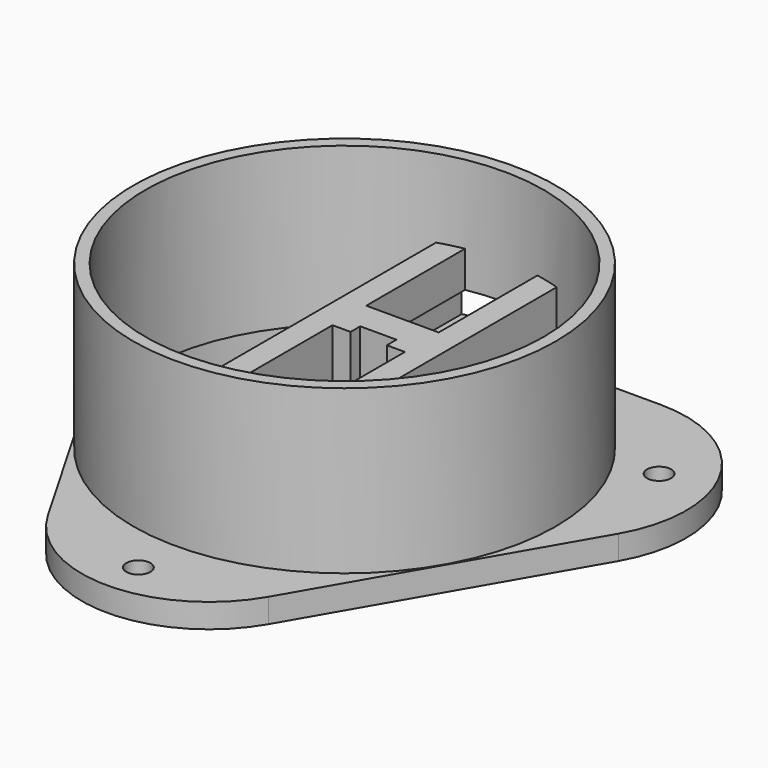
from build123d import *

# Parameters (mm, degrees)
F0_R              = 35
F0_R_2            = 33
F2_DEPTH          = 31
F3_DEPTH          = 18
F4_E28_W          = 6
F4_E28_H          = 7.5
F4_E39_MIRRORCS_W = 6
F4_E39_MIRRORCS_H = 7.5
F5_DEPTH          = 9.3
F7_DEPTH          = 4
F8_R              = 21.1
F9_R              = 2
F10_DEPTH         = 38
F11_DEPTH         = 52
F12_DEPTH         = 37.9
F13_R             = 33.8752288108
F14_DEPTH         = 4.9
F15_W             = 4.2938441038
F15_H             = 3.1884626523
F16_DEPTH         = 17.2


with BuildPart() as f2:
    # F0 (on Top) → F2 (new body)
    with BuildSketch(Plane.XY):
        Circle(F0_R)
        Circle(F0_R_2, mode=Mode.SUBTRACT)
    extrude(amount=F2_DEPTH)

    # F1 (on Top) → F3 (join)
    with BuildSketch(Plane.XY):
        Polygon((10, -32.0528298616), (10, -24), (10, 32.2797112167), (6, 33.4707275033), (6, 12), (3, 12), (0, 12), (-3, 12), (-6, 12), (-6, 33.4707275033), (-10, 32.2797112167), (-10, -24), (-10, -32.0528298616), (-6, -33.1044308841), (-6, -24), (0, -24), (6, -24), (6, -33.1044308841), align=None)
        Polygon((0, 7), (3, 7), (3, 5), (6, 5), (6, -19), (0, -19), (-6, -19), (-6, 5), (-3, 5), (-3, 7), align=None, mode=Mode.SUBTRACT)
    extrude(amount=F3_DEPTH)

    # F4_E28 (on explicit) + F4_E39_MirrorCS (on explicit) → F5 (cut)
    with BuildSketch(Plane.XZ.offset(24)):
        with Locations((3, 3.75)):
            Rectangle(F4_E28_W, F4_E28_H)
    with BuildSketch(Plane(origin=(0, -24, 0), x_dir=(-1, 0, 0), z_dir=(0, 1, 0))):
        with Locations((3, 3.75)):
            Rectangle(F4_E39_MIRRORCS_W, F4_E39_MIRRORCS_H)
    extrude(amount=-F5_DEPTH, dir=(0, -1, 0), mode=Mode.SUBTRACT)

    # F6 (on Top) → F7 (join)
    with BuildSketch(Plane.XY):
        Polygon((60.8495350583, 35.131495446), (-60.8495350583, 35.131495446), (0, -70.2629908919), align=None)
    extrude(amount=F7_DEPTH)

    # F8
    f8_edges = [f2.edges().sort_by_distance(p)[0] for p in [
        (-60.849535, 35.131495, 2),
        (60.849535, 35.131495, 2),
        (0, -70.262991, 2),
    ]]
    fillet(f8_edges, radius=F8_R)

    # F9 (on Top) → F10 (cut)
    with BuildSketch(Plane.XY):
        with Locations((-37.2817739844, 20.93468979)):
            Circle(F9_R)
        with Locations((0, -42.7055284381)):
            Circle(F9_R)
        with Locations((36.2159647048, 19.8873784393)):
            Circle(F9_R)
    extrude(amount=-F10_DEPTH, mode=Mode.SUBTRACT)

    # F9 (on Top) → F11 (cut)
    with BuildSketch(Plane.XY):
        with Locations((36.2159647048, 19.8873784393)):
            Circle(F9_R)
    extrude(amount=F11_DEPTH, mode=Mode.SUBTRACT)

    # F9 (on Top) → F12 (cut)
    with BuildSketch(Plane.XY):
        with Locations((-37.2817739844, 20.93468979)):
            Circle(F9_R)
        with Locations((0, -42.7055284381)):
            Circle(F9_R)
    extrude(amount=F12_DEPTH, mode=Mode.SUBTRACT)

    # F13 (on Top) → F14 (cut)
    with BuildSketch(Plane.XY):
        Circle(F13_R)
    extrude(amount=F14_DEPTH, mode=Mode.SUBTRACT)

    # F15 (on face) → F16 (cut)
    with BuildSketch(Plane(origin=(0, 35.131495446, 0), x_dir=(-1, 0, 0), z_dir=(0, 1, 0))):
        Polygon((-7.865479216, 7.1884626523), (-0.6682581179, 7.1884626523), (0.0053993426, 7.1884626523), (0.0053993426, 10.3769253045), (4.2992434464, 10.3769253045), (4.2992434464, 7.1884626523), (7.865479216, 7.1884626523), (7.865479216, 11.9928242639), (-7.865479216, 11.9928242639), align=None)
        with Locations((2.1523213945, 8.7826939784)):
            Rectangle(F15_W, F15_H)
        with Locations((2.1523213945, 5.5942313261)):
            Rectangle(F15_W, F15_H)
    extrude(amount=-F16_DEPTH, mode=Mode.SUBTRACT)


solid = f2.part
